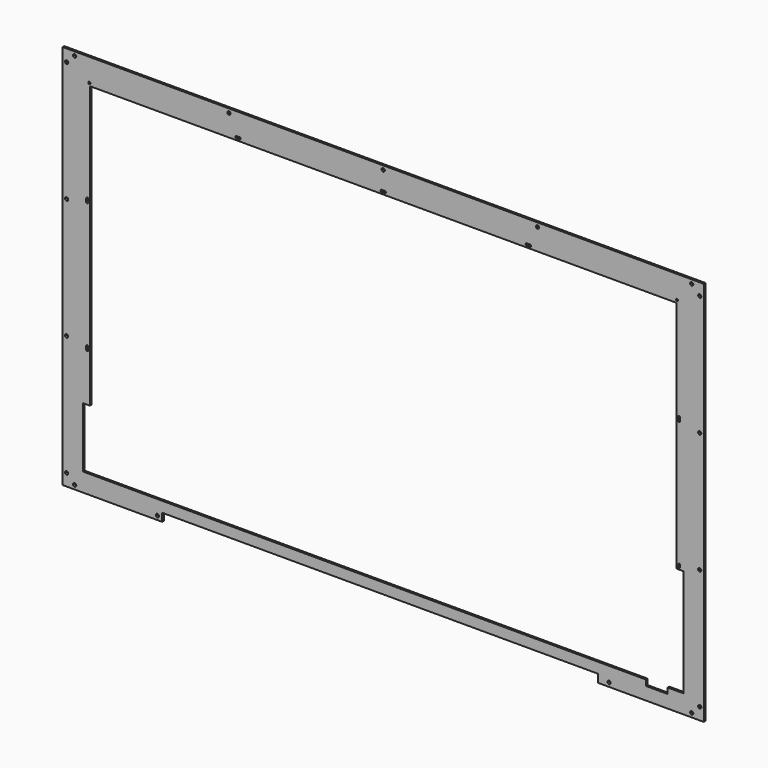
from build123d import *

# Parameters (mm, degrees)
F0_R     = 5.969
F0_R_2   = 1.75
F1_DEPTH = 1.5875


# Not quite as in the source:
# - a feature names something its author has since deleted; it is built from what else it names


with BuildPart() as f1:
    # F0 (on Front) → F1 (new body, symmetric)
    with BuildSketch(Plane.XZ):
        Polygon((495.3, -292.89375), (495.3, 292.89375), (-495.3, 292.89375), (-495.3, -292.89375), (-350.29902, -292.89375), (340.29904, -292.89375), align=None)
        Polygon((-475.996, -180.775), (-475.996, 276.225), (0, 276.225), (230, 276.225), (465.646, 276.225), (475.996, 276.225), (475.996, 104.225), (475.996, -101.775), (475.996, -105.775), (475.996, -276.225), (450.596, -276.225), (450.596, -285.225), (416.596, -285.225), (416.596, -276.225), (-475.996, -276.225), align=None, mode=Mode.SUBTRACT)
        Polygon((-495.3, 292.89375), (495.3, 292.89375), (495.3, -292.89375), (340.29904, -292.89375), (340.29904, -305.59375), (508, -305.59375), (508, 305.59375), (-508, 305.59375), align=None)
        Polygon((357.84, -296.70375), (360.38, -296.70375), (360.38, -299.24375), (360.38, -301.78375), (357.84, -301.78375), (355.3, -301.78375), (355.3, -299.24375), (355.3, -296.70375), align=None, mode=Mode.SUBTRACT)
        Polygon((486.41, -299.24375), (486.41, -296.70375), (488.95, -296.70375), (491.49, -296.70375), (491.49, -299.24375), (491.49, -301.78375), (488.95, -301.78375), (486.41, -301.78375), align=None, mode=Mode.SUBTRACT)
        Polygon((501.65, -289.08375), (499.11, -289.08375), (499.11, -286.54375), (499.11, -284.00375), (501.65, -284.00375), (504.19, -284.00375), (504.19, -286.54375), (504.19, -289.08375), align=None, mode=Mode.SUBTRACT)
        Polygon((501.65, -98.0545833333), (499.11, -98.0545833333), (499.11, -95.5145833333), (499.11, -92.9745833333), (501.65, -92.9745833333), (504.19, -92.9745833333), (504.19, -95.5145833333), (504.19, -98.0545833333), align=None, mode=Mode.SUBTRACT)
        with Locations((-488.95, 299.24375)):
            Circle(F0_R, mode=Mode.SUBTRACT)
        Polygon((-244.475, 301.78375), (-241.935, 301.78375), (-241.935, 299.24375), (-241.935, 296.70375), (-244.475, 296.70375), (-247.015, 296.70375), (-247.015, 299.24375), (-247.015, 301.78375), align=None, mode=Mode.SUBTRACT)
        Polygon((504.19, 95.5145833333), (504.19, 92.9745833333), (501.65, 92.9745833333), (499.11, 92.9745833333), (499.11, 95.5145833333), (499.11, 98.0545833333), (501.6500000218, 98.0545833333), (504.19, 98.0545833333), align=None, mode=Mode.SUBTRACT)
        Polygon((0, 301.78375), (2.54, 301.78375), (2.54, 299.24375), (2.54, 296.70375), (0, 296.70375), (-2.54, 296.70375), (-2.54, 299.24375), (-2.54, 301.78375), align=None, mode=Mode.SUBTRACT)
        Polygon((244.475, 296.70375), (241.935, 296.70375), (241.935, 299.24375), (241.935, 301.78375), (244.475, 301.78375), (247.015, 301.78375), (247.015, 299.24375), (247.015, 296.70375), align=None, mode=Mode.SUBTRACT)
        Polygon((501.65, 284.00375), (499.11, 284.00375), (499.11, 286.54375), (499.11, 289.08375), (501.65, 289.08375), (504.19, 289.08375), (504.19, 286.54375), (504.19, 284.00375), align=None, mode=Mode.SUBTRACT)
        Polygon((486.41, 299.24375), (486.41, 301.78375), (488.95, 301.78375), (491.49, 301.78375), (491.49, 299.24375), (491.49, 296.70375), (488.95, 296.70375), (486.41, 296.70375), align=None, mode=Mode.SUBTRACT)
        Polygon((-495.3, -292.89375), (-495.3, 292.89375), (-508, 305.59375), (-508, -305.59375), (-350.29902, -305.59375), (-350.29902, -292.89375), align=None)
        Polygon((-486.41, -299.24375), (-486.41, -301.78375), (-488.95, -301.78375), (-491.49, -301.78375), (-491.49, -299.24375), (-491.49, -296.70375), (-488.95, -296.70375), (-486.41, -296.70375), align=None, mode=Mode.SUBTRACT)
        Polygon((-504.19, -284.00375), (-501.65, -284.00375), (-499.11, -284.00375), (-499.11, -286.54375), (-499.11, -289.08375), (-501.65, -289.08375), (-504.19, -289.08375), (-504.19, -286.54375), align=None, mode=Mode.SUBTRACT)
        Polygon((-357.84, -296.70375), (-355.3, -296.70375), (-355.3, -299.24375), (-355.3, -301.78375), (-357.84, -301.78375), (-360.38, -301.78375), (-360.38, -299.24375), (-360.38, -296.70375), align=None, mode=Mode.SUBTRACT)
        Polygon((-504.19, -92.9745833333), (-501.65, -92.9745833333), (-499.11, -92.9745833333), (-499.11, -95.5145833333), (-499.11, -98.0545833333), (-501.65, -98.0545833333), (-504.19, -98.0545833333), (-504.19, -95.5145833333), align=None, mode=Mode.SUBTRACT)
        Polygon((-504.19, 98.0545833333), (-501.65, 98.0545833333), (-499.11, 98.0545833333), (-499.11, 95.5145833333), (-499.11, 92.9745833333), (-501.65, 92.9745833333), (-504.19, 92.9745833333), (-504.19, 95.5145833333), align=None, mode=Mode.SUBTRACT)
        Polygon((-501.65, 284.00375), (-504.19, 284.00375), (-504.19, 286.54375), (-504.19, 289.08375), (-501.65, 289.08375), (-499.11, 289.08375), (-499.11, 286.54375), (-499.11, 284.00375), align=None, mode=Mode.SUBTRACT)
        Polygon((0, 276.225), (-475.996, 276.225), (-475.996, -180.775), (-464.79587, -180.775), (-464.79587, 265.02614), (464.79587, 265.02614), (464.79587, -105.775), (475.996, -105.775), (475.996, -101.775), (475.996, 104.225), (475.996, 276.225), (465.646, 276.225), (230, 276.225), align=None)
        with BuildLine():
            Line((-467.246, -99.275), (-467.246, -101.775))
            Line((-467.246, -101.775), (-467.246, -104.275))
            ThreePointArc((-467.246, -104.275), (-468.996, -106.025), (-470.746, -104.275))
            Line((-470.746, -104.275), (-470.746, -101.775))
            Line((-470.746, -101.775), (-470.746, -99.275))
            ThreePointArc((-470.746, -99.275), (-468.996, -97.525), (-467.246, -99.275))
        make_face(mode=Mode.SUBTRACT)
        with BuildLine():
            Line((470.746, -99.275), (470.746, -101.775))
            ThreePointArc((470.746, -101.775), (470.2334368671, -103.0124368671), (468.996, -103.525))
            ThreePointArc((468.996, -103.525), (467.7585631329, -103.0124368671), (467.246, -101.775))
            Line((467.246, -101.775), (467.246, -99.275))
            ThreePointArc((467.246, -99.275), (468.996, -97.525), (470.746, -99.275))
        make_face(mode=Mode.SUBTRACT)
        with BuildLine():
            Line((-467.246, 106.725), (-467.246, 104.225))
            Line((-467.246, 104.225), (-467.246, 101.725))
            ThreePointArc((-467.246, 101.725), (-468.996, 99.975), (-470.746, 101.725))
            Line((-470.746, 101.725), (-470.746, 104.225))
            Line((-470.746, 104.225), (-470.746, 106.725))
            ThreePointArc((-470.746, 106.725), (-468.996, 108.475), (-467.246, 106.725))
        make_face(mode=Mode.SUBTRACT)
        with Locations((-465.646, 269.225)):
            Circle(F0_R_2, mode=Mode.SUBTRACT)
        with BuildLine():
            Line((-232.5, 270.975), (-230, 270.975))
            Line((-230, 270.975), (-227.5, 270.975))
            ThreePointArc((-227.5, 270.975), (-225.75, 269.225), (-227.5, 267.475))
            Line((-227.5, 267.475), (-230, 267.475))
            Line((-230, 267.475), (-232.5, 267.475))
            ThreePointArc((-232.5, 267.475), (-234.25, 269.225), (-232.5, 270.975))
        make_face(mode=Mode.SUBTRACT)
        with BuildLine():
            Line((470.746, 106.725), (470.746, 104.225))
            Line((470.746, 104.225), (470.746, 101.725))
            ThreePointArc((470.746, 101.725), (468.996, 99.975), (467.246, 101.725))
            Line((467.246, 101.725), (467.246, 104.225))
            Line((467.246, 104.225), (467.246, 106.725))
            ThreePointArc((467.246, 106.725), (468.996, 108.475), (470.746, 106.725))
        make_face(mode=Mode.SUBTRACT)
        with BuildLine():
            Line((-2.5, 270.975), (0, 270.975))
            Line((0, 270.975), (2.5, 270.975))
            ThreePointArc((2.5, 270.975), (4.25, 269.225), (2.5, 267.475))
            Line((2.5, 267.475), (0, 267.475))
            Line((0, 267.475), (-2.5, 267.475))
            ThreePointArc((-2.5, 267.475), (-4.25, 269.225), (-2.5, 270.975))
        make_face(mode=Mode.SUBTRACT)
        with BuildLine():
            Line((227.5, 270.975), (230, 270.975))
            Line((230, 270.975), (232.5, 270.975))
            ThreePointArc((232.5, 270.975), (234.25, 269.225), (232.5, 267.475))
            Line((232.5, 267.475), (230, 267.475))
            Line((230, 267.475), (227.5, 267.475))
            ThreePointArc((227.5, 267.475), (225.75, 269.225), (227.5, 270.975))
        make_face(mode=Mode.SUBTRACT)
        with BuildLine():
            ThreePointArc((467.396, 269.225), (464.4085631329, 267.9875631329), (465.646, 270.975))
            ThreePointArc((465.646, 270.975), (466.8834368671, 270.4624368671), (467.396, 269.225))
        make_face(mode=Mode.SUBTRACT)
        with Locations((-488.95, 299.24375)):
            Circle(F0_R)
        Polygon((-486.41, 299.24375), (-486.41, 296.70375), (-488.95, 296.70375), (-491.49, 296.70375), (-491.49, 299.24375), (-491.49, 301.78375), (-488.95, 301.78375), (-486.41, 301.78375), align=None, mode=Mode.SUBTRACT)
        with BuildLine():
            ThreePointArc((488.95, 296.70375), (487.1539487758, 297.4476987758), (486.41, 299.24375))
            Line((486.41, 299.24375), (486.41, 296.70375))
            Line((486.41, 296.70375), (488.95, 296.70375))
        make_face()
        with BuildLine():
            Line((488.95, 301.78375), (486.41, 301.78375))
            Line((486.41, 301.78375), (486.41, 299.24375))
            ThreePointArc((486.41, 299.24375), (487.1539487758, 301.0398012242), (488.95, 301.78375))
        make_face()
        with BuildLine():
            Line((491.49, 301.78375), (488.95, 301.78375))
            ThreePointArc((488.95, 301.78375), (490.7460512242, 301.0398012242), (491.49, 299.24375))
            Line((491.49, 299.24375), (491.49, 301.78375))
        make_face()
        with BuildLine():
            Line((491.49, 296.70375), (491.49, 299.24375))
            ThreePointArc((491.49, 299.24375), (490.7460512242, 297.4476987758), (488.95, 296.70375))
            Line((488.95, 296.70375), (491.49, 296.70375))
        make_face()
        with BuildLine():
            Line((499.11, 289.08375), (499.11, 286.54375))
            ThreePointArc((499.11, 286.54375), (499.8539487758, 288.3398012242), (501.65, 289.08375))
            Line((501.65, 289.08375), (499.11, 289.08375))
        make_face()
        with BuildLine():
            Line((504.19, 289.08375), (501.65, 289.08375))
            ThreePointArc((501.65, 289.08375), (503.4460512242, 288.3398012242), (504.19, 286.54375))
            Line((504.19, 286.54375), (504.19, 289.08375))
        make_face()
        with BuildLine():
            ThreePointArc((504.19, 286.54375), (503.4460512242, 284.7476987758), (501.65, 284.00375))
            Line((501.65, 284.00375), (504.19, 284.00375))
            Line((504.19, 284.00375), (504.19, 286.54375))
        make_face()
        with BuildLine():
            Line((499.11, 286.54375), (499.11, 284.00375))
            Line((499.11, 284.00375), (501.65, 284.00375))
            ThreePointArc((501.65, 284.00375), (499.8539487758, 284.7476987758), (499.11, 286.54375))
        make_face()
        with BuildLine():
            ThreePointArc((244.475, 301.78375), (246.2710512242, 301.0398012242), (247.015, 299.24375))
            Line((247.015, 299.24375), (247.015, 301.78375))
            Line((247.015, 301.78375), (244.475, 301.78375))
        make_face()
        with BuildLine():
            Line((241.935, 301.78375), (241.935, 299.24375))
            ThreePointArc((241.935, 299.24375), (242.6789487758, 301.0398012242), (244.475, 301.78375))
            Line((244.475, 301.78375), (241.935, 301.78375))
        make_face()
        with BuildLine():
            Line((241.935, 299.24375), (241.935, 296.70375))
            Line((241.935, 296.70375), (244.475, 296.70375))
            ThreePointArc((244.475, 296.70375), (242.6789487758, 297.4476987758), (241.935, 299.24375))
        make_face()
        with BuildLine():
            ThreePointArc((247.015, 299.24375), (246.2710512242, 297.4476987758), (244.475, 296.70375))
            Line((244.475, 296.70375), (247.015, 296.70375))
            Line((247.015, 296.70375), (247.015, 299.24375))
        make_face()
        with BuildLine():
            ThreePointArc((-2.54, 299.24375), (-1.7960512242, 301.0398012242), (0, 301.78375))
            Line((0, 301.78375), (-2.54, 301.78375))
            Line((-2.54, 301.78375), (-2.54, 299.24375))
        make_face()
        with BuildLine():
            ThreePointArc((0, 296.70375), (-1.7960512242, 297.4476987758), (-2.54, 299.24375))
            Line((-2.54, 299.24375), (-2.54, 296.70375))
            Line((-2.54, 296.70375), (0, 296.70375))
        make_face()
        with BuildLine():
            Line((2.54, 296.70375), (2.54, 299.24375))
            ThreePointArc((2.54, 299.24375), (1.7960512242, 297.4476987758), (0, 296.70375))
            Line((0, 296.70375), (2.54, 296.70375))
        make_face()
        with BuildLine():
            Line((2.54, 299.24375), (2.54, 301.78375))
            Line((2.54, 301.78375), (0, 301.78375))
            ThreePointArc((0, 301.78375), (1.7960512242, 301.0398012242), (2.54, 299.24375))
        make_face()
        with BuildLine():
            Line((-241.935, 299.24375), (-241.935, 301.78375))
            Line((-241.935, 301.78375), (-244.475, 301.78375))
            ThreePointArc((-244.475, 301.78375), (-242.6789487758, 301.0398012242), (-241.935, 299.24375))
        make_face()
        with BuildLine():
            ThreePointArc((-247.015, 299.24375), (-246.2710512242, 301.0398012242), (-244.475, 301.78375))
            Line((-244.475, 301.78375), (-247.015, 301.78375))
            Line((-247.015, 301.78375), (-247.015, 299.24375))
        make_face()
        with BuildLine():
            ThreePointArc((-244.475, 296.70375), (-246.2710512242, 297.4476987758), (-247.015, 299.24375))
            Line((-247.015, 299.24375), (-247.015, 296.70375))
            Line((-247.015, 296.70375), (-244.475, 296.70375))
        make_face()
        with BuildLine():
            Line((-241.935, 296.70375), (-241.935, 299.24375))
            ThreePointArc((-241.935, 299.24375), (-242.6789487758, 297.4476987758), (-244.475, 296.70375))
            Line((-244.475, 296.70375), (-241.935, 296.70375))
        make_face()
        with BuildLine():
            Line((-491.49, 301.78375), (-491.49, 299.24375))
            ThreePointArc((-491.49, 299.24375), (-490.7460512242, 301.0398012242), (-488.95, 301.78375))
            Line((-488.95, 301.78375), (-491.49, 301.78375))
        make_face()
        with BuildLine():
            ThreePointArc((-488.95, 301.78375), (-487.1539487758, 301.0398012242), (-486.41, 299.24375))
            Line((-486.41, 299.24375), (-486.41, 301.78375))
            Line((-486.41, 301.78375), (-488.95, 301.78375))
        make_face()
        with BuildLine():
            Line((-488.95, 296.70375), (-486.41, 296.70375))
            Line((-486.41, 296.70375), (-486.41, 299.24375))
            ThreePointArc((-486.41, 299.24375), (-487.1539487758, 297.4476987758), (-488.95, 296.70375))
        make_face()
        with BuildLine():
            Line((-491.49, 296.70375), (-488.95, 296.70375))
            ThreePointArc((-488.95, 296.70375), (-490.7460512242, 297.4476987758), (-491.49, 299.24375))
            Line((-491.49, 299.24375), (-491.49, 296.70375))
        make_face()
        with BuildLine():
            Line((-499.11, 289.08375), (-501.65, 289.08375))
            ThreePointArc((-501.65, 289.08375), (-499.8539487758, 288.3398012242), (-499.11, 286.54375))
            Line((-499.11, 286.54375), (-499.11, 289.08375))
        make_face()
        with BuildLine():
            Line((-504.19, 289.08375), (-504.19, 286.54375))
            ThreePointArc((-504.19, 286.54375), (-503.4460512242, 288.3398012242), (-501.65, 289.08375))
            Line((-501.65, 289.08375), (-504.19, 289.08375))
        make_face()
        with BuildLine():
            Line((-504.19, 286.54375), (-504.19, 284.00375))
            Line((-504.19, 284.00375), (-501.65, 284.00375))
            ThreePointArc((-501.65, 284.00375), (-503.4460512242, 284.7476987758), (-504.19, 286.54375))
        make_face()
        with BuildLine():
            ThreePointArc((-499.11, 286.54375), (-499.8539487758, 284.7476987758), (-501.65, 284.00375))
            Line((-501.65, 284.00375), (-499.11, 284.00375))
            Line((-499.11, 284.00375), (-499.11, 286.54375))
        make_face()
        with BuildLine():
            Line((-499.11, 98.0545833333), (-501.65, 98.0545833333))
            ThreePointArc((-501.65, 98.0545833333), (-499.8539487758, 97.3106345575), (-499.11, 95.5145833333))
            Line((-499.11, 95.5145833333), (-499.11, 98.0545833333))
        make_face()
        with BuildLine():
            ThreePointArc((-504.19, 95.5145833333), (-503.4460512242, 97.3106345575), (-501.65, 98.0545833333))
            Line((-501.65, 98.0545833333), (-504.19, 98.0545833333))
            Line((-504.19, 98.0545833333), (-504.19, 95.5145833333))
        make_face()
        with BuildLine():
            Line((-499.11, 92.9745833333), (-499.11, 95.5145833333))
            ThreePointArc((-499.11, 95.5145833333), (-499.8539487758, 93.7185321091), (-501.65, 92.9745833333))
            Line((-501.65, 92.9745833333), (-499.11, 92.9745833333))
        make_face()
        with BuildLine():
            ThreePointArc((-501.65, 92.9745833333), (-503.4460512242, 93.7185321091), (-504.19, 95.5145833333))
            Line((-504.19, 95.5145833333), (-504.19, 92.9745833333))
            Line((-504.19, 92.9745833333), (-501.65, 92.9745833333))
        make_face()
        with BuildLine():
            Line((-499.11, -92.9745833333), (-501.65, -92.9745833333))
            ThreePointArc((-501.65, -92.9745833333), (-499.8539487758, -93.7185321091), (-499.11, -95.5145833333))
            Line((-499.11, -95.5145833333), (-499.11, -92.9745833333))
        make_face()
        with BuildLine():
            ThreePointArc((-504.19, -95.5145833333), (-503.4460512242, -93.7185321091), (-501.65, -92.9745833333))
            Line((-501.65, -92.9745833333), (-504.19, -92.9745833333))
            Line((-504.19, -92.9745833333), (-504.19, -95.5145833333))
        make_face()
        with BuildLine():
            Line((-499.11, -98.0545833333), (-499.11, -95.5145833333))
            ThreePointArc((-499.11, -95.5145833333), (-499.8539487758, -97.3106345575), (-501.65, -98.0545833333))
            Line((-501.65, -98.0545833333), (-499.11, -98.0545833333))
        make_face()
        with BuildLine():
            ThreePointArc((-501.65, -98.0545833333), (-503.4460512242, -97.3106345575), (-504.19, -95.5145833333))
            Line((-504.19, -95.5145833333), (-504.19, -98.0545833333))
            Line((-504.19, -98.0545833333), (-501.65, -98.0545833333))
        make_face()
        with BuildLine():
            Line((-499.11, -284.00375), (-501.65, -284.00375))
            ThreePointArc((-501.65, -284.00375), (-499.8539487758, -284.7476987758), (-499.11, -286.54375))
            Line((-499.11, -286.54375), (-499.11, -284.00375))
        make_face()
        with BuildLine():
            ThreePointArc((-504.19, -286.54375), (-503.4460512242, -284.7476987758), (-501.65, -284.00375))
            Line((-501.65, -284.00375), (-504.19, -284.00375))
            Line((-504.19, -284.00375), (-504.19, -286.54375))
        make_face()
        with BuildLine():
            ThreePointArc((-501.65, -289.08375), (-503.4460512242, -288.3398012242), (-504.19, -286.54375))
            Line((-504.19, -286.54375), (-504.19, -289.08375))
            Line((-504.19, -289.08375), (-501.65, -289.08375))
        make_face()
        with BuildLine():
            Line((-499.11, -289.08375), (-499.11, -286.54375))
            ThreePointArc((-499.11, -286.54375), (-499.8539487758, -288.3398012242), (-501.65, -289.08375))
            Line((-501.65, -289.08375), (-499.11, -289.08375))
        make_face()
        with BuildLine():
            Line((-491.49, -296.70375), (-491.49, -299.24375))
            ThreePointArc((-491.49, -299.24375), (-490.7460512242, -297.4476987758), (-488.95, -296.70375))
            Line((-488.95, -296.70375), (-491.49, -296.70375))
        make_face()
        with BuildLine():
            ThreePointArc((-488.95, -296.70375), (-487.1539487758, -297.4476987758), (-486.41, -299.24375))
            Line((-486.41, -299.24375), (-486.41, -296.70375))
            Line((-486.41, -296.70375), (-488.95, -296.70375))
        make_face()
        with BuildLine():
            Line((-488.95, -301.78375), (-486.41, -301.78375))
            Line((-486.41, -301.78375), (-486.41, -299.24375))
            ThreePointArc((-486.41, -299.24375), (-487.1539487758, -301.0398012242), (-488.95, -301.78375))
        make_face()
        with BuildLine():
            Line((-491.49, -301.78375), (-488.95, -301.78375))
            ThreePointArc((-488.95, -301.78375), (-490.7460512242, -301.0398012242), (-491.49, -299.24375))
            Line((-491.49, -299.24375), (-491.49, -301.78375))
        make_face()
        with BuildLine():
            Line((-355.3, -299.24375), (-355.3, -296.70375))
            Line((-355.3, -296.70375), (-357.84, -296.70375))
            ThreePointArc((-357.84, -296.70375), (-356.0439487758, -297.4476987758), (-355.3, -299.24375))
        make_face()
        with BuildLine():
            ThreePointArc((-360.38, -299.24375), (-359.6360512242, -297.4476987758), (-357.84, -296.70375))
            Line((-357.84, -296.70375), (-360.38, -296.70375))
            Line((-360.38, -296.70375), (-360.38, -299.24375))
        make_face()
        with BuildLine():
            ThreePointArc((-357.84, -301.78375), (-359.6360512242, -301.0398012242), (-360.38, -299.24375))
            Line((-360.38, -299.24375), (-360.38, -301.78375))
            Line((-360.38, -301.78375), (-357.84, -301.78375))
        make_face()
        with BuildLine():
            Line((-355.3, -301.78375), (-355.3, -299.24375))
            ThreePointArc((-355.3, -299.24375), (-356.0439487758, -301.0398012242), (-357.84, -301.78375))
            Line((-357.84, -301.78375), (-355.3, -301.78375))
        make_face()
        with BuildLine():
            Line((360.38, -299.24375), (360.38, -296.70375))
            Line((360.38, -296.70375), (357.84, -296.70375))
            ThreePointArc((357.84, -296.70375), (359.6360512242, -297.4476987758), (360.38, -299.24375))
        make_face()
        with BuildLine():
            ThreePointArc((355.3, -299.24375), (356.0439487758, -297.4476987758), (357.84, -296.70375))
            Line((357.84, -296.70375), (355.3, -296.70375))
            Line((355.3, -296.70375), (355.3, -299.24375))
        make_face()
        with BuildLine():
            Line((355.3, -301.78375), (357.84, -301.78375))
            ThreePointArc((357.84, -301.78375), (356.0439487758, -301.0398012242), (355.3, -299.24375))
            Line((355.3, -299.24375), (355.3, -301.78375))
        make_face()
        with BuildLine():
            Line((360.38, -301.78375), (360.38, -299.24375))
            ThreePointArc((360.38, -299.24375), (359.6360512242, -301.0398012242), (357.84, -301.78375))
            Line((357.84, -301.78375), (360.38, -301.78375))
        make_face()
        with BuildLine():
            Line((491.49, -296.70375), (488.95, -296.70375))
            ThreePointArc((488.95, -296.70375), (490.7460512242, -297.4476987758), (491.49, -299.24375))
            Line((491.49, -299.24375), (491.49, -296.70375))
        make_face()
        with BuildLine():
            Line((488.95, -296.70375), (486.41, -296.70375))
            Line((486.41, -296.70375), (486.41, -299.24375))
            ThreePointArc((486.41, -299.24375), (487.1539487758, -297.4476987758), (488.95, -296.70375))
        make_face()
        with BuildLine():
            ThreePointArc((488.95, -301.78375), (487.1539487758, -301.0398012242), (486.41, -299.24375))
            Line((486.41, -299.24375), (486.41, -301.78375))
            Line((486.41, -301.78375), (488.95, -301.78375))
        make_face()
        with BuildLine():
            ThreePointArc((491.49, -299.24375), (490.7460512242, -301.0398012242), (488.95, -301.78375))
            Line((488.95, -301.78375), (491.49, -301.78375))
            Line((491.49, -301.78375), (491.49, -299.24375))
        make_face()
        with BuildLine():
            ThreePointArc((501.65, -284.00375), (503.4460512242, -284.7476987758), (504.19, -286.54375))
            Line((504.19, -286.54375), (504.19, -284.00375))
            Line((504.19, -284.00375), (501.65, -284.00375))
        make_face()
        with BuildLine():
            Line((499.11, -284.00375), (499.11, -286.54375))
            ThreePointArc((499.11, -286.54375), (499.8539487758, -284.7476987758), (501.65, -284.00375))
            Line((501.65, -284.00375), (499.11, -284.00375))
        make_face()
        with BuildLine():
            Line((499.11, -286.54375), (499.11, -289.08375))
            Line((499.11, -289.08375), (501.65, -289.08375))
            ThreePointArc((501.65, -289.08375), (499.8539487758, -288.3398012242), (499.11, -286.54375))
        make_face()
        with BuildLine():
            ThreePointArc((504.19, -286.54375), (503.4460512242, -288.3398012242), (501.65, -289.08375))
            Line((501.65, -289.08375), (504.19, -289.08375))
            Line((504.19, -289.08375), (504.19, -286.54375))
        make_face()
        with BuildLine():
            ThreePointArc((501.6500000218, 98.0545833333), (503.4460512319, 97.3106345499), (504.19, 95.5145833333))
            Line((504.19, 95.5145833333), (504.19, 98.0545833333))
            Line((504.19, 98.0545833333), (501.6500000218, 98.0545833333))
        make_face()
        with BuildLine():
            Line((499.11, 98.0545833333), (499.11, 95.5145833333))
            ThreePointArc((499.11, 95.5145833333), (499.8539487835, 97.3106345652), (501.6500000218, 98.0545833333))
            Line((501.6500000218, 98.0545833333), (499.11, 98.0545833333))
        make_face()
        with BuildLine():
            Line((499.11, 92.9745833333), (501.65, 92.9745833333))
            ThreePointArc((501.65, 92.9745833333), (499.8539487758, 93.7185321091), (499.11, 95.5145833333))
            Line((499.11, 95.5145833333), (499.11, 92.9745833333))
        make_face()
        with BuildLine():
            Line((501.65, 92.9745833333), (504.19, 92.9745833333))
            Line((504.19, 92.9745833333), (504.19, 95.5145833333))
            ThreePointArc((504.19, 95.5145833333), (503.4460512242, 93.7185321091), (501.65, 92.9745833333))
        make_face()
        with BuildLine():
            ThreePointArc((501.65, -92.9745833333), (503.4460512242, -93.7185321091), (504.19, -95.5145833333))
            Line((504.19, -95.5145833333), (504.19, -92.9745833333))
            Line((504.19, -92.9745833333), (501.65, -92.9745833333))
        make_face()
        with BuildLine():
            Line((499.11, -92.9745833333), (499.11, -95.5145833333))
            ThreePointArc((499.11, -95.5145833333), (499.8539487758, -93.7185321091), (501.65, -92.9745833333))
            Line((501.65, -92.9745833333), (499.11, -92.9745833333))
        make_face()
        with BuildLine():
            Line((499.11, -95.5145833333), (499.11, -98.0545833333))
            Line((499.11, -98.0545833333), (501.65, -98.0545833333))
            ThreePointArc((501.65, -98.0545833333), (499.8539487758, -97.3106345575), (499.11, -95.5145833333))
        make_face()
        with BuildLine():
            ThreePointArc((504.19, -95.5145833333), (503.4460512242, -97.3106345575), (501.65, -98.0545833333))
            Line((501.65, -98.0545833333), (504.19, -98.0545833333))
            Line((504.19, -98.0545833333), (504.19, -95.5145833333))
        make_face()
    extrude(amount=F1_DEPTH, both=True)


solid = f1.part
